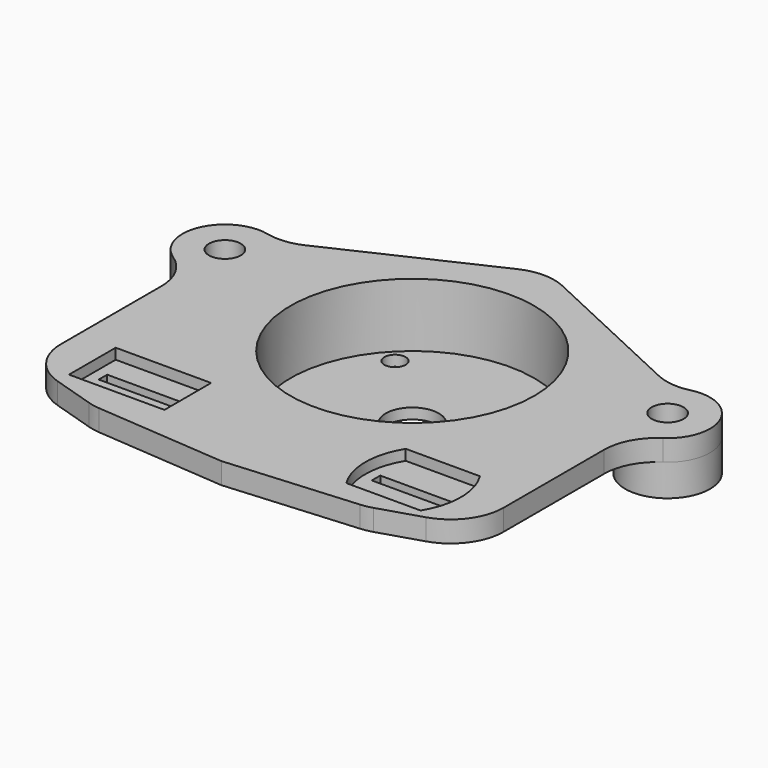
from build123d import *
from build123d import SkipClean  # not in build123d's __all__

# Parameters (mm, degrees)
F0_R      = 13.5
F0_R_2    = 1
F0_R_3    = 2.5
F1_DEPTH  = 1
F2_R      = 13.5
F2_R_2    = 11.5
F3_DEPTH  = 6
F4_W      = 7
F4_H      = 1
F4_R      = 1.5
F4_R_2    = 13.5
F5_DEPTH  = 2
F6_R      = 5
F7_W      = 7
F7_H      = 7
F7_W_2    = 9
F7_H_2    = 5.5
F8_DEPTH  = 1
F9_R      = 4
F9_R_2    = 1.5
F10_DEPTH = 3


with BuildPart() as f1:
    # F0 (on Top) → F1 (new body)
    with BuildSketch(Plane.XY):
        Circle(F0_R)
        with Locations((7.1922094223, -6.9478143056)):
            Circle(F0_R_2, mode=Mode.SUBTRACT)
        with Locations((-7.1922094223, 6.9478143056)):
            Circle(F0_R_2, mode=Mode.SUBTRACT)
        Circle(F0_R_3, mode=Mode.SUBTRACT)
    extrude(amount=F1_DEPTH)

    # F2 (on face) → F3 (join)
    with BuildSketch(Plane.XY.offset(1)):
        Circle(F2_R)
        Circle(F2_R_2, mode=Mode.SUBTRACT)
    extrude(amount=F3_DEPTH)

    # F4 (on face) → F5 (join)
    with BuildSketch(Plane.XY.offset(7)):
        with BuildLine():
            Line((-12.875, -21.5), (0, -22.5089902885))
            Line((0, -22.5089902885), (12.875, -21.5))
            Line((12.875, -21.5), (20.875, -19))
            Line((20.875, -19), (20.875, 0))
            ThreePointArc((20.875, 0), (24.6990897298, 5.1731742149), (18.6318382667, 7.3118311307))
            Line((18.6318382667, 7.3118311307), (0, 16))
            Line((0, 16), (-18.6318382667, 7.3118311307))
            ThreePointArc((-18.6318382667, 7.3118311307), (-24.6990897298, 5.1731742149), (-20.875, 0))
            Line((-20.875, 0), (-20.875, -19))
            Line((-20.875, -19), (-12.875, -21.5))
        make_face()
        with Locations((-12.875, -16)):
            Rectangle(F4_W, F4_H, mode=Mode.SUBTRACT)
        with Locations((12.875, -16)):
            Rectangle(F4_W, F4_H, mode=Mode.SUBTRACT)
        with Locations((-20.875, 4)):
            Circle(F4_R, mode=Mode.SUBTRACT)
        Circle(F4_R_2, mode=Mode.SUBTRACT)
        with Locations((20.875, 4)):
            Circle(F4_R, mode=Mode.SUBTRACT)
    extrude(amount=-F5_DEPTH)

    # F6
    f6_edges = [f1.edges().sort_by_distance(p)[0] for p in [
        (0, 16, 6),
        (20.875, -19, 6),
        (12.875, -21.5, 6),
        (-12.875, -21.5, 6),
        (-20.875, -19, 6),
        (-20.875, 0, 6),
        (-18.631838, 7.311831, 6),
        (18.631838, 7.311831, 6),
        (20.875, 0, 6),
    ]]
    fillet(f6_edges, radius=F6_R)

    # F7 (on face) → F8 (cut)
    with BuildSketch(Plane.XY.offset(7)):
        with Locations((12.875, -16)):
            Rectangle(F7_W, F7_H)
        with BuildLine():
            ThreePointArc((16.375, -19.5), (17.375, -16), (16.375, -12.5))
            Line((16.375, -12.5), (16.375, -19.5))
        make_face()
        with BuildLine():
            Line((9.375, -19.5), (9.375, -12.5))
            ThreePointArc((9.375, -12.5), (8.375, -16), (9.375, -19.5))
        make_face()
        with Locations((-12.875, -16)):
            Rectangle(F7_W_2, F7_H_2)
    extrude(amount=-F8_DEPTH, mode=Mode.SUBTRACT)

    # F9 (on face) → F10 (join)
    with BuildSketch(Plane(origin=(0, 0, 5), x_dir=(1, 0, 0), z_dir=(0, 0, -1))):
        with Locations((20.875, -4)):
            Circle(F9_R)
        with Locations((20.875, -4)):
            Circle(F9_R_2, mode=Mode.SUBTRACT)
        with Locations((-20.875, -4)):
            Circle(F9_R)
        with Locations((-20.875, -4)):
            Circle(F9_R_2, mode=Mode.SUBTRACT)
    with SkipClean():  # cleaning this boolean's faces spoils the solid; the shape is the same uncleaned
        extrude(amount=F10_DEPTH)


solid = f1.part
